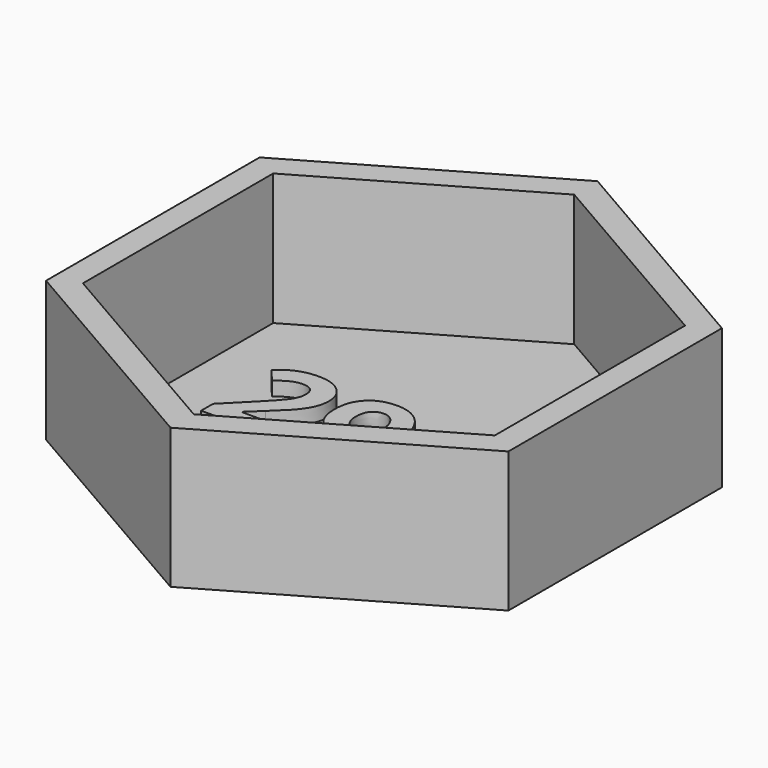
from build123d import *

# Parameters (mm, degrees)
F2_DEPTH     = 10
F4_DEPTH     = 25
F5_TEXT_SIZE = 10.1156067103
F6_DEPTH     = 1


# Not quite as in the source:
# - Text() gives the source's letters only with a copy of the font that has no kerning and outlines rounded to 1/6400 em; it was checked with that copy


with BuildPart() as f2:
    # F1 (on offset) → F2 (new body)
    with BuildSketch(Plane.XY.offset(-0.6)):
        Polygon((0, -19.0525588833), (16.5, -9.5262794416), (16.5, 9.5262794416), (0, 19.0525588833), (-16.5, 9.5262794416), (-16.5, -9.5262794416), align=None)
    extrude(amount=F2_DEPTH)

    # F3 (on Top) → F4 (cut)
    with BuildSketch(Plane.XY):
        Polygon((-14.7, -8.4870489571), (0, -16.9740979142), (14.7, -8.4870489571), (14.7, 8.4870489571), (0, 16.9740979142), (-14.7, 8.4870489571), align=None)
    extrude(amount=F4_DEPTH, mode=Mode.SUBTRACT)


with BuildPart() as f6:
    # F5 (on Top) → F6 (new body)
    with BuildSketch(Plane.XY):
        with Locations((-10.4323702567, -3.782828222)):
            Text('29.4', F5_TEXT_SIZE, font='Open Sans', font_style=FontStyle.BOLD, text_align=(TextAlign.LEFT, TextAlign.BOTTOM))
    extrude(amount=F6_DEPTH)


solid = Compound([f2.part, f6.part])
